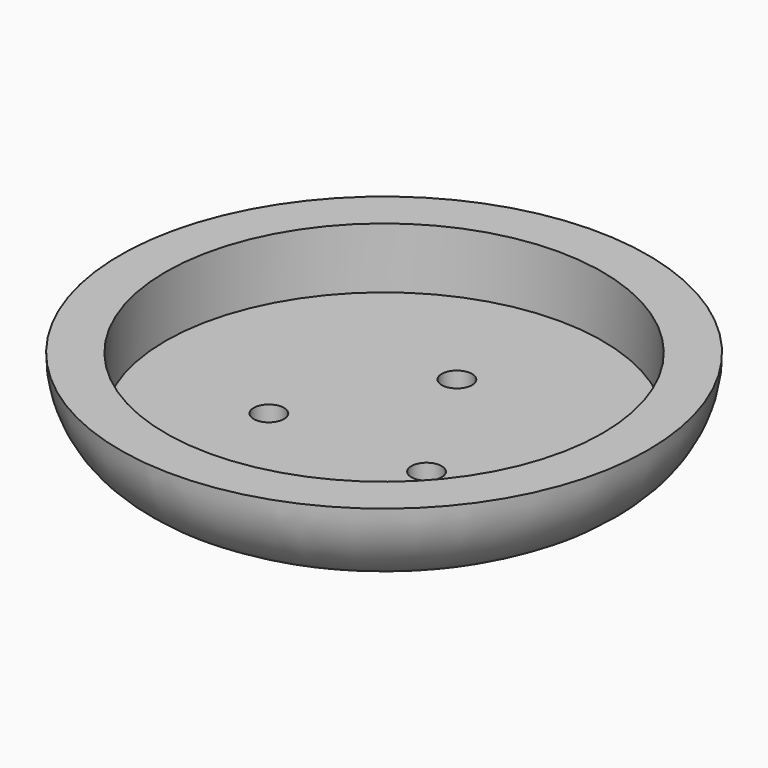
from build123d import *

# Parameters (mm, degrees)
F2_R           = 14.99999
F4_D           = 5
F4_CBORE_D     = 8
F4_CBORE_DEPTH = 2


# Not quite as in the source:
# - a fillet or chamfer is up to 0.001 mm smaller than in the source, because OpenCascade refuses the exact size


with BuildPart() as f1:
    # F0 (on Front) → F1 (revolve)
    with BuildSketch(Plane.XZ):
        Polygon((36, -25), (0, -25), (0, -30), (43.5, -30), (43.5, -15), (36, -15), align=None)
    revolve(axis=Axis((0, 0, -27.5), (0, 0, 1)))

    # F2 (radius 15 in the source; OpenCascade refuses exactly that, so slightly less here)
    f2_edges = [f1.edges().sort_by_distance(p)[0] for p in [
        (-43.5, 0, -30),
    ]]
    fillet(f2_edges, radius=F2_R)

    # F4 (through all)
    with Locations(Plane(origin=(0, 0, -30), x_dir=(1, 0, 0), z_dir=(0, 0, -1))):
        with Locations((-12.9903810568, 7.5), (12.9903810568, 7.5), (0, -15)):
            CounterBoreHole(F4_D / 2, F4_CBORE_D / 2, F4_CBORE_DEPTH)


solid = f1.part
